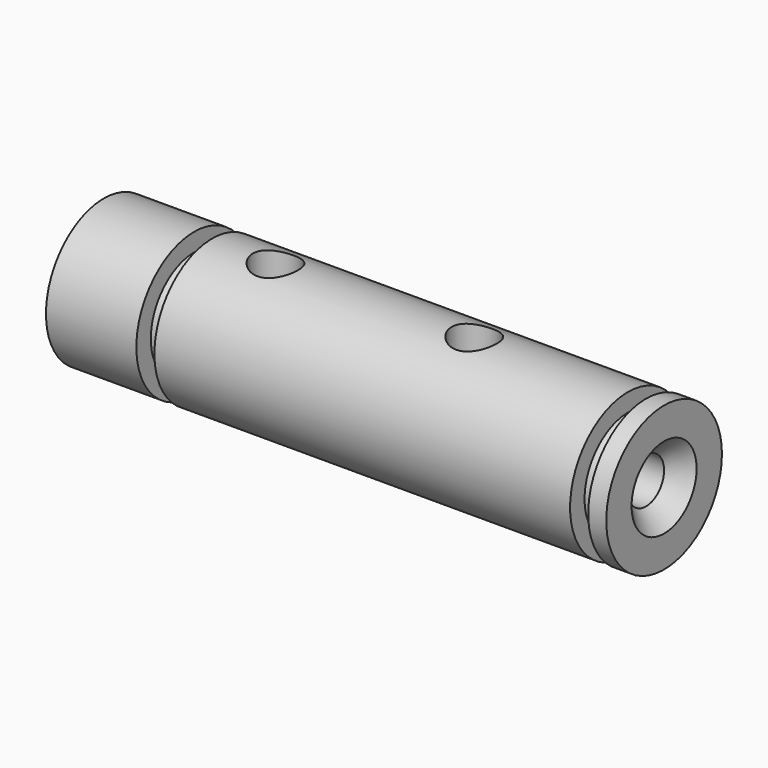
from build123d import *

# Parameters (mm, degrees)
F3_R     = 1.25
F4_DEPTH = 25
F5_SIZE  = 1
F8_DEPTH = 2


with BuildPart() as f1:
    # F0 (on Top) → F1 (revolve)
    with BuildSketch(Plane.XY):
        Polygon((0, 1.25), (0, 2.9657871928), (0, 4), (-1, 4), (-1, 3), (-2, 3), (-2, 4), (-3, 4), (-8, 4), (-13, 4), (-19, 4), (-24, 4), (-25, 4), (-25, 3), (-26, 3), (-26, 4), (-31, 4), (-31, 1), (-27, 1), (-27, 0), (-5, 0), (-5, 1.25), (-0.9906101976, 1.25), align=None)
    revolve(axis=Axis((5.4950757935, 0, 0), (1, 0, 0)))

    # F3 (on offset) → F4 (cut)
    with BuildSketch(Plane.XY.offset(4)):
        with Locations((-21.5, 0)):
            Circle(F3_R)
        with Locations((-10.5, 0)):
            Circle(F3_R)
    extrude(amount=-F4_DEPTH, mode=Mode.SUBTRACT)

    # F5
    f5_edges = [f1.edges().sort_by_distance(p)[0] for p in [
        (0, -1.25, 0),
    ]]
    chamfer(f5_edges, length=F5_SIZE)

    # F7 (on offset) → F8 (cut)
    with BuildSketch(Plane.XZ.offset(-4)):
        with BuildLine():
            Line((-21.5, -1.25), (-10.5, -1.25))
            ThreePointArc((-10.5, -1.25), (-9.25, 0), (-10.5, 1.25))
            Line((-10.5, 1.25), (-21.5, 1.25))
            ThreePointArc((-21.5, 1.25), (-22.75, 0), (-21.5, -1.25))
        make_face()
    extrude(amount=F8_DEPTH, mode=Mode.SUBTRACT)


solid = f1.part
